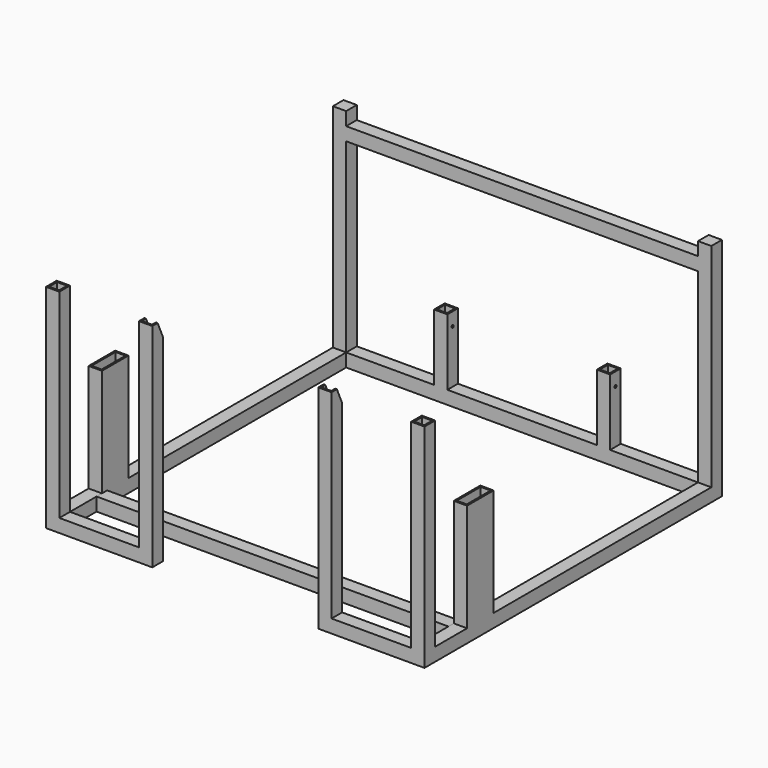
from build123d import *

# Parameters (mm, degrees)
F0_W      = 723.9
F0_H      = 711.2
F0_W_2    = 673.1
F0_H_2    = 660.4
F1_DEPTH  = 25.4
F2_W      = 25.4
F2_H      = 25.4
F3_DEPTH  = 381
F4_W      = 25.4
F4_H      = 25.4
F5_DEPTH  = 381
F6_W      = 673.1
F6_H      = 25.4
F7_DEPTH  = 25.4
F8_W      = 317.5
F8_H      = 25.4
F9_DEPTH  = 25.4
F10_T     = -3.175
F11_W     = 25.4
F11_H     = 25.4
F12_DEPTH = 406.4
F13_W     = 25.4
F13_H     = 25.4
F14_DEPTH = 673.1
F15_W     = 25.4
F15_H     = 63.3782297373
F15_W_2   = 19.05
F15_H_2   = 57.0282297373
F16_DEPTH = 206.375
F17_W     = 25.4
F17_H     = 25.4
F17_W_2   = 19.05
F17_H_2   = 19.05
F18_DEPTH = 127
F20_D     = 5.1054
F20_DEPTH = 406.4
F20_TIP   = 1.5338169022
F22_DEPTH = 406.4


# Not quite as in the source:
# - a pattern or mirror of a feature is missing from the dataset's text; its kind, count and spacing are read off the source's solid


with BuildPart() as f1:
    # F0 (on Top) → F1 (new body)
    with BuildSketch(Plane.XY):
        Rectangle(F0_W, F0_H)
        Rectangle(F0_W_2, F0_H_2, mode=Mode.SUBTRACT)
    extrude(amount=F1_DEPTH)

    # F2 (on face) → F3 (join)
    with BuildSketch(Plane.XY.offset(25.4)):
        with Locations((-349.25, -342.9)):
            Rectangle(F2_W, F2_H)
        with Locations((349.25, -342.9)):
            Rectangle(F2_W, F2_H)
    extrude(amount=F3_DEPTH)

    # F4 (on face) → F5 (join)
    with BuildSketch(Plane.XY.offset(25.4)):
        with Locations((-171.45, -342.9)):
            Rectangle(F4_W, F4_H)
        with Locations((171.45, -342.9)):
            Rectangle(F4_W, F4_H)
    extrude(amount=F5_DEPTH)

    # F8 (on face) → F9 (cut)
    with BuildSketch(Plane.XY.offset(25.4)):
        with Locations((0, -342.9)):
            Rectangle(F8_W, F8_H)
    extrude(amount=-F9_DEPTH, mode=Mode.SUBTRACT)

    # F10
    f10_openings = [f1.faces().sort_by_distance(p)[0] for p in [
        (-349.25, -342.9, 406.4),
        (-171.45, -342.9, 406.4),
        (171.45, -342.9, 406.4),
        (349.25, -342.9, 406.4),
    ]]
    offset(amount=F10_T, openings=f10_openings, kind=Kind.INTERSECTION)

    # F11 (on face) → F12 (join)
    with BuildSketch(Plane.XY.offset(25.4)):
        with Locations((349.25, 342.9)):
            Rectangle(F11_W, F11_H)
        with Locations((-349.25, 342.9)):
            Rectangle(F11_W, F11_H)
    extrude(amount=F12_DEPTH)

    # F13 (on face) → F14 (join)
    with BuildSketch(Plane.YZ.offset(-336.55)):
        with Locations((342.9, 393.7)):
            Rectangle(F13_W, F13_H)
    extrude(amount=F14_DEPTH)

    # F15 (on face) → F16 (join)
    with BuildSketch(Plane.XY.offset(25.4)):
        with Locations((349.25, -222.1086844802)):
            Rectangle(F15_W, F15_H)
        with Locations((349.25, -222.1086844802)):
            Rectangle(F15_W_2, F15_H_2, mode=Mode.SUBTRACT)
    f16 = extrude(amount=F16_DEPTH)

    # F16_copies: F16 across plane
    add(f16.mirror(Plane(origin=(0, 0, 0), x_dir=(0, 0, -1), z_dir=(-1, 0, 0))))

    # F17 (on face) → F18 (join)
    with BuildSketch(Plane.XY.offset(25.4)):
        with Locations((-155.702, 342.9)):
            Rectangle(F17_W, F17_H)
        with Locations((-155.702, 342.9)):
            Rectangle(F17_W_2, F17_H_2, mode=Mode.SUBTRACT)
        with Locations((155.702, 342.9)):
            Rectangle(F17_W, F17_H)
        with Locations((155.702, 342.9)):
            Rectangle(F17_W_2, F17_H_2, mode=Mode.SUBTRACT)
    extrude(amount=F18_DEPTH)

    # F20 (one way)
    with BuildSketch(Plane.YZ.offset(168.402)):
        with Locations((342.9, 127)):
            Circle(F20_D / 2)
    extrude(amount=-F20_DEPTH, mode=Mode.SUBTRACT)
    with Locations(Plane.YZ.offset(168.402)):
        with Locations((342.9, 127)):
            with Locations((0, 0, -(F20_DEPTH + F20_TIP / 2))):  # 118° drill point
                Cone(0, F20_D / 2, F20_TIP, mode=Mode.SUBTRACT)

    # F21 (on face) → F22 (cut)
    with BuildSketch(Plane.YZ.offset(184.15)):
        Polygon((-351.5427708626, 424.6743917465), (-342.9, 406.4), (-303.1188249588, 316.628485918), (-308.5665404797, 412.8710329533), align=None)
    extrude(amount=-F22_DEPTH, mode=Mode.SUBTRACT)


with BuildPart() as f7:
    # F6 (on face) → F7 (new body)
    with BuildSketch(Plane.XY.offset(25.4)):
        with Locations((0, -254)):
            Rectangle(F6_W, F6_H)
    extrude(amount=-F7_DEPTH)


solid = Compound([f1.part, f7.part])
